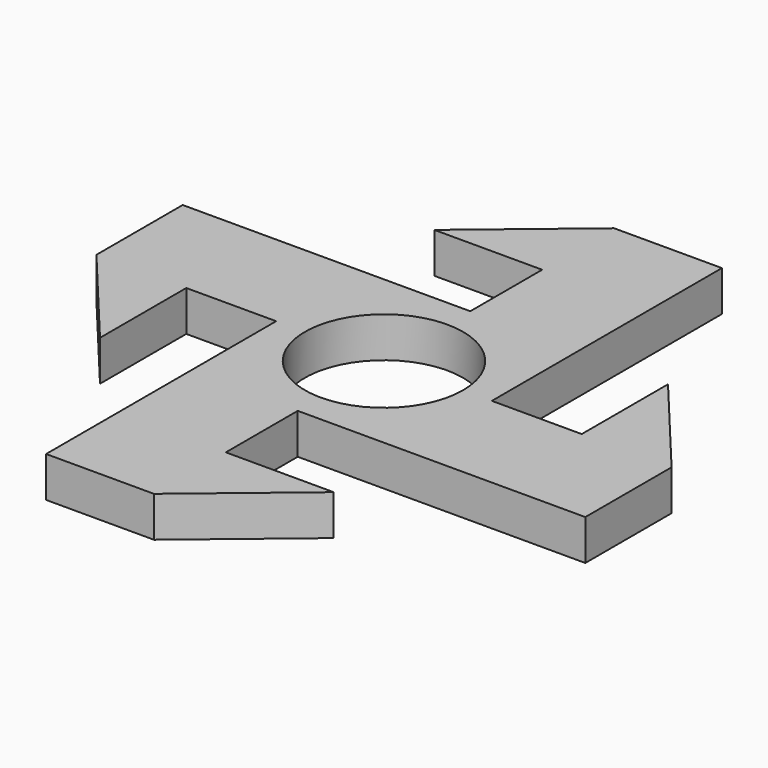
from build123d import *

# Parameters (mm, degrees)
F0_R     = 11.176
F1_DEPTH = 5.715
F2_DEPTH = 5.715


# Not quite as in the source:
# - a feature names something its author has since deleted; it is built from what else it names


with BuildPart() as f1:
    # F0 (on Top) → F1 (new body)
    with BuildSketch(Plane.XY):
        with BuildLine():
            ThreePointArc((0, -15.24), (10.7763073453, -10.7763073453), (15.24, 0))
            ThreePointArc((15.24, 0), (10.7763073453, 10.7763073453), (0, 15.24))
            ThreePointArc((0, 15.24), (-10.7763073453, 10.7763073453), (-15.24, 0))
            ThreePointArc((-15.24, 0), (-10.7763073453, -10.7763073453), (0, -15.24))
        make_face()
        Circle(F0_R, mode=Mode.SUBTRACT)
        with BuildLine():
            Line((27.94, 0), (15.24, 0))
            ThreePointArc((15.24, 0), (10.7763073453, -10.7763073453), (0, -15.24))
            Line((0, -15.24), (40.64, -15.24))
            Line((40.64, -15.24), (40.64, 0))
            Line((40.64, 0), (27.94, 0))
        make_face()
        with BuildLine():
            ThreePointArc((0, 15.24), (10.7763073453, 10.7763073453), (15.24, 0))
            Line((15.24, 0), (15.24, 40.64))
            Line((15.24, 40.64), (0, 40.64))
            Line((0, 40.64), (0, 27.94))
            Line((0, 27.94), (0, 15.24))
        make_face()
        with BuildLine():
            ThreePointArc((-15.24, 0), (-10.7763073453, 10.7763073453), (0, 15.24))
            Line((0, 15.24), (-40.64, 15.24))
            Line((-40.64, 15.24), (-40.64, 0))
            Line((-40.64, 0), (-27.94, 0))
            Line((-27.94, 0), (-15.24, 0))
        make_face()
        with BuildLine():
            Line((0, -27.94), (0, -15.24))
            ThreePointArc((0, -15.24), (-10.7763073453, -10.7763073453), (-15.24, 0))
            Line((-15.24, 0), (-15.24, -40.64))
            Line((-15.24, -40.64), (0, -40.64))
            Line((0, -40.64), (0, -27.94))
        make_face()
    extrude(amount=F1_DEPTH)

    # F0 (on Top) → F2 (join)
    with BuildSketch(Plane.XY):
        with BuildLine():
            ThreePointArc((0, -15.24), (10.7763073453, -10.7763073453), (15.24, 0))
            ThreePointArc((15.24, 0), (10.7763073453, 10.7763073453), (0, 15.24))
            ThreePointArc((0, 15.24), (-10.7763073453, 10.7763073453), (-15.24, 0))
            ThreePointArc((-15.24, 0), (-10.7763073453, -10.7763073453), (0, -15.24))
        make_face()
        Circle(F0_R, mode=Mode.SUBTRACT)
        with BuildLine():
            Line((27.94, 0), (15.24, 0))
            ThreePointArc((15.24, 0), (10.7763073453, -10.7763073453), (0, -15.24))
            Line((0, -15.24), (40.64, -15.24))
            Line((40.64, -15.24), (40.64, 0))
            Line((40.64, 0), (27.94, 0))
        make_face()
        with BuildLine():
            ThreePointArc((0, 15.24), (10.7763073453, 10.7763073453), (15.24, 0))
            Line((15.24, 0), (15.24, 40.64))
            Line((15.24, 40.64), (0, 40.64))
            Line((0, 40.64), (0, 27.94))
            Line((0, 27.94), (0, 15.24))
        make_face()
        with BuildLine():
            ThreePointArc((-15.24, 0), (-10.7763073453, 10.7763073453), (0, 15.24))
            Line((0, 15.24), (-40.64, 15.24))
            Line((-40.64, 15.24), (-40.64, 0))
            Line((-40.64, 0), (-27.94, 0))
            Line((-27.94, 0), (-15.24, 0))
        make_face()
        with BuildLine():
            Line((0, -27.94), (0, -15.24))
            ThreePointArc((0, -15.24), (-10.7763073453, -10.7763073453), (-15.24, 0))
            Line((-15.24, 0), (-15.24, -40.64))
            Line((-15.24, -40.64), (0, -40.64))
            Line((0, -40.64), (0, -27.94))
        make_face()
        Polygon((27.94, 15.24), (27.94, 0), (40.64, 0), align=None)
        Polygon((-15.24, 27.94), (0, 27.94), (0, 40.64), align=None)
        Polygon((15.24, -27.94), (0, -27.94), (0, -40.64), align=None)
        Polygon((-27.94, -15.24), (-27.94, 0), (-40.64, 0), align=None)
    extrude(amount=F2_DEPTH)


solid = f1.part
